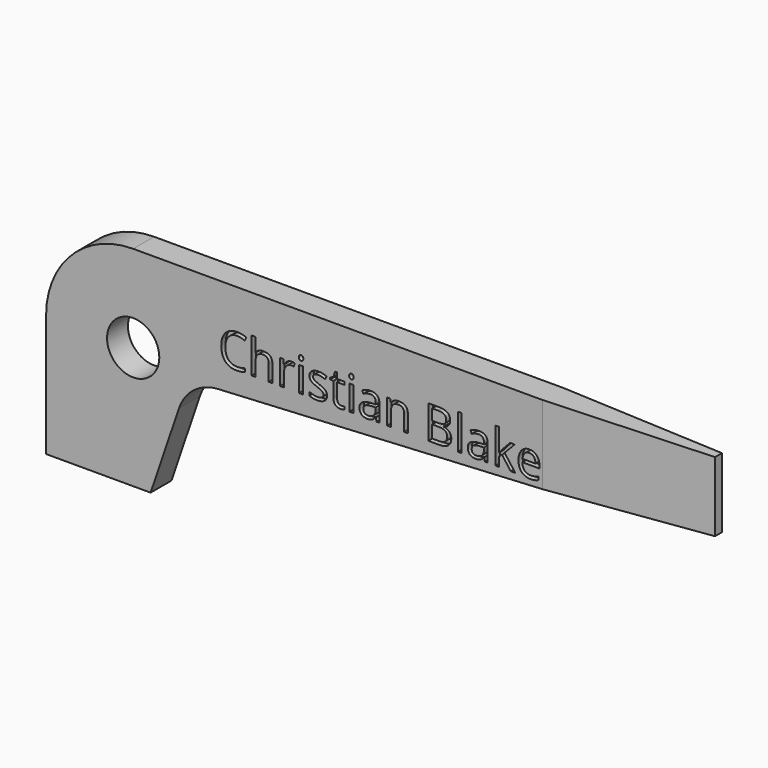
from build123d import *

# Parameters (mm, degrees)
F1_DEPTH     = 2.38125
F2_R         = 2.38125
F3_DEPTH     = 2.38225
F5_DEPTH     = 25.4
F6_TEXT_SIZE = 4.2355961064
F7_DEPTH     = 0.508


# Not quite as in the source:
# - Text() gives the source's letters only with a copy of the font that has no kerning and outlines rounded to 1/6400 em; it was checked with that copy


with BuildPart() as f1:
    # F0 (on Front) → F1 (new body)
    with BuildSketch(Plane.XZ):
        with BuildLine():
            Line((60.325, 19.05), (7.9375, 19.05))
            ThreePointArc((7.9375, 19.05), (2.3248399243, 16.7251600757), (0, 11.1125))
            Line((0, 11.1125), (0, 0))
            Line((0, 0), (9.525, 0))
            Line((9.525, 0), (12.1173647876, 7.6271664624))
            ThreePointArc((12.1173647876, 7.6271664624), (13.4786145605, 9.5135918491), (15.6631963617, 10.3130942181))
            Line((15.6631963617, 10.3130942181), (60.325, 12.7))
            Line((60.325, 12.7), (60.325, 19.05))
        make_face()
    extrude(amount=F1_DEPTH)

    # F2 (on face) → F3 (cut, through all)
    with BuildSketch(Plane.XZ.offset(2.38125)):
        with Locations((7.9375, 11.1125)):
            Circle(F2_R)
    extrude(amount=-F3_DEPTH, mode=Mode.SUBTRACT)

    # F4 (on face) → F5 (cut)
    with BuildSketch(Plane.XY.offset(19.05)):
        Polygon((60.325, 0), (45.24375, 0), (60.325, -0.79375), align=None)
        Polygon((60.325, -2.38125), (60.325, -1.5875), (45.24375, -2.38125), align=None)
    extrude(amount=-F5_DEPTH, mode=Mode.SUBTRACT)

    # F6 (on face) → F7 (cut)
    with BuildSketch(Plane.XZ.offset(2.38125)):
        with Locations((15.7044380295, 12.3901549577)):
            Text('Christian Blake', F6_TEXT_SIZE, font='Open Sans', text_align=(TextAlign.LEFT, TextAlign.BOTTOM))
    extrude(amount=-F7_DEPTH, mode=Mode.SUBTRACT)


solid = f1.part
